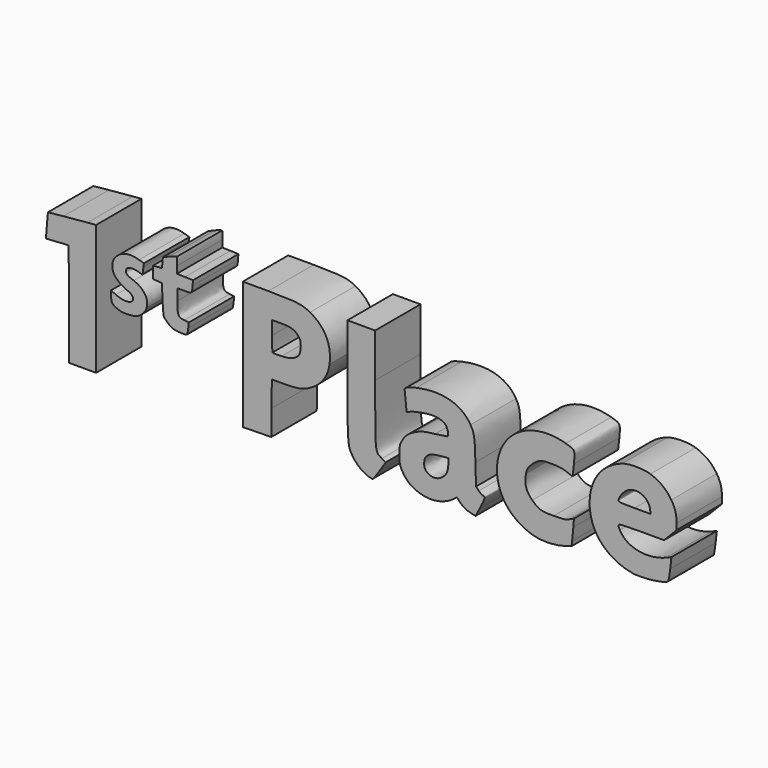
from build123d import *

# Parameters (mm, degrees)
F1_DEPTH = 6.35


# Not quite as in the source:
# - ends of sketch curves that miss each other by under 0.0002 mm in the source are joined


with BuildPart() as f1:
    # F0 (on Front) → F1 (new body)
    with BuildSketch(Plane.XZ):
        with BuildLine():
            add(Edge.make_bspline(
                [(0.3341400629, -8.891573857), (-0.294670775, -8.6645318704), (-0.976808264, -8.1246552902), (-1.3296902624, -7.574737026)],
                knots=[0, 0, 0, 0, 1, 1, 1, 1], degree=3))
            add(Edge.make_bspline(
                [(0.8350588344, -9.0026580356), (0.7635369283, -9.0152123713), (0.5381243175, -8.9652247697), (0.3341400629, -8.891573857)],
                knots=[0, 0, 0, 0, 1, 1, 1, 1], degree=3))
            add(Edge.make_bspline(
                [(1.6370563807, -7.9375592211), (1.2674791345, -8.510809568), (0.9065796253, -8.9901037), (0.8350588344, -9.0026580356)],
                knots=[0, 0, 0, 0, 1, 1, 1, 1], degree=3))
            Line((1.6370563807, -7.9375592211), (1.8985483475, -6.6505150987))
            add(Edge.make_bspline(
                [(1.123237547, 0.7960059272), (1.123237547, -6.5406989559), (1.0841035293, -6.1648384081), (1.8985483475, -6.6505150987)],
                knots=[0, 0, 0, 0, 1, 1, 1, 1], degree=3))
            Line((1.123237547, 0.7960059272), (1.1249048919, 5.7024196408))
            Line((1.1249048919, 5.7024196408), (-1.9611174698, 5.7063939098))
            Line((-1.9611174698, 5.7063939098), (-1.9611174698, 0.6585863056))
            add(Edge.make_bspline(
                [(-1.3296902624, -7.574737026), (-1.9722420587, -6.5734069203), (-1.9611174698, -6.7184604076), (-1.9611174698, 0.6585863056)],
                knots=[0, 0, 0, 0, 1, 1, 1, 1], degree=3))
        make_face()
        Polygon((1.8985483475, -6.6505150987), (1.6370563807, -7.9375592211), (2.3090161255, -6.8952883976), align=None)
    extrude(amount=F1_DEPTH)


with BuildPart() as f1b:
    # F0 (on Front) → F1, piece 2 (new body)
    with BuildSketch(Plane.XZ):
        with BuildLine():
            add(Edge.make_bspline(
                [(6.6803148923, -8.8230898838), (5.4982367035, -8.6125914713), (4.6605144496, -8.0535092224), (4.1522941559, -7.135933052)],
                knots=[0, 0, 0, 0, 1, 1, 1, 1], degree=3))
            add(Edge.make_bspline(
                [(9.910150536, -8.0284407), (9.0040190305, -8.7195815781), (7.78427895, -9.0196789355), (6.6803148923, -8.8230898838)],
                knots=[0, 0, 0, 0, 1, 1, 1, 1], degree=3))
            Line((9.910150536, -8.0284407), (10.2834750122, -7.7436924873))
            Line((10.2834750122, -7.7436924873), (10.5754578323, -8.0633735822))
            add(Edge.make_bspline(
                [(11.9336714428, -8.8088994808), (11.3485816335, -8.6774375088), (10.9229141541, -8.4437876836), (10.5754578323, -8.0633735822)],
                knots=[0, 0, 0, 0, 1, 1, 1, 1], degree=3))
            Line((11.9336714428, -8.8088994808), (12.3629088279, -8.9053426966))
            Line((12.3629088279, -8.9053426966), (12.8352650082, -8.0015967045))
            add(Edge.make_bspline(
                [(13.2301672836, -6.6273569945), (13.4991191377, -6.6273569945), (13.4326637987, -6.8586134996), (12.8352650082, -8.0015967045)],
                knots=[0, 0, 0, 0, 1, 1, 1, 1], degree=3))
            add(Edge.make_bspline(
                [(12.7221990357, -6.3069833312), (12.8910965041, -6.4831890133), (13.1196819926, -6.6273569945), (13.2301672836, -6.6273569945)],
                knots=[0, 0, 0, 0, 1, 1, 1, 1], degree=3))
            Line((12.7221990357, -6.3069833312), (12.4151135405, -5.9866096679))
            Line((12.4151135405, -5.9866096679), (12.3465570762, -3.6147078996))
            add(Edge.make_bspline(
                [(11.7983451399, -0.1012894763), (12.2270594741, -0.8328368689), (12.2750385158, -1.1403271987), (12.3465570762, -3.6147078996)],
                knots=[0, 0, 0, 0, 1, 1, 1, 1], degree=3))
            add(Edge.make_bspline(
                [(5.7503494429, 1.5688051915), (8.5603079697, 2.2020480209), (10.8130600929, 1.5799721598), (11.7983451399, -0.1012894763)],
                knots=[0, 0, 0, 0, 1, 1, 1, 1], degree=3))
            add(Edge.make_bspline(
                [(4.6961912015, 1.2469192532), (4.858749606, 1.3299315493), (5.3331199224, 1.4747798312), (5.7503494429, 1.5688051915)],
                knots=[0, 0, 0, 0, 1, 1, 1, 1], degree=3))
            add(Edge.make_bspline(
                [(4.4566316824, 0.7107497541), (4.4067221482, 1.0541008516), (4.4327698574, 1.1124015044), (4.6961912015, 1.2469192532)],
                knots=[0, 0, 0, 0, 1, 1, 1, 1], degree=3))
            add(Edge.make_bspline(
                [(4.5795397099, -0.4295992373), (4.5427399042, -0.0142890569), (4.4874303439, 0.4988684354), (4.4566316824, 0.7107497541)],
                knots=[0, 0, 0, 0, 1, 1, 1, 1], degree=3))
            Line((4.5795397099, -0.4295992373), (4.6464489543, -1.184710684))
            Line((4.6464489543, -1.184710684), (5.0072993927, -1.03393821))
            add(Edge.make_bspline(
                [(7.5522841514, -0.5632013683), (6.849403068, -0.5632013683), (5.5656132364, -0.8006586468), (5.0072993927, -1.03393821)],
                knots=[0, 0, 0, 0, 1, 1, 1, 1], degree=3))
            add(Edge.make_bspline(
                [(9.0299909029, -1.0454040645), (8.7617907253, -0.7334761668), (8.2399856077, -0.5632013683), (7.5522841514, -0.5632013683)],
                knots=[0, 0, 0, 0, 1, 1, 1, 1], degree=3))
            add(Edge.make_bspline(
                [(9.222734583, -2.0813848949), (9.3763431301, -1.986449493), (9.2485547818, -1.2996045464), (9.0299909029, -1.0454040645)],
                knots=[0, 0, 0, 0, 1, 1, 1, 1], degree=3))
            add(Edge.make_bspline(
                [(7.8341817928, -2.2987833406), (8.5349439069, -2.2181130633), (9.1597933874, -2.1202835954), (9.222734583, -2.0813848949)],
                knots=[0, 0, 0, 0, 1, 1, 1, 1], degree=3))
            add(Edge.make_bspline(
                [(5.5145226556, -2.8919966091), (6.2193665737, -2.5260584139), (6.5136646466, -2.4507959693), (7.8341817928, -2.2987833406)],
                knots=[0, 0, 0, 0, 1, 1, 1, 1], degree=3))
            add(Edge.make_bspline(
                [(4.1460398507, -4.1437375873), (4.462187843, -3.573149335), (4.8030229433, -3.2613887243), (5.5145226556, -2.8919966091)],
                knots=[0, 0, 0, 0, 1, 1, 1, 1], degree=3))
            add(Edge.make_bspline(
                [(3.841652138, -5.6340901247), (3.841652138, -4.7904213738), (3.8731333307, -4.6362819691), (4.1460398507, -4.1437375873)],
                knots=[0, 0, 0, 0, 1, 1, 1, 1], degree=3))
            add(Edge.make_bspline(
                [(4.1522941559, -7.135933052), (3.872362695, -6.6305265265), (3.841652138, -6.4820503461), (3.841652138, -5.6340901247)],
                knots=[0, 0, 0, 0, 1, 1, 1, 1], degree=3))
        make_face()
        with BuildLine():
            add(Edge.make_bspline(
                [(8.4953860954, -6.3921090203), (9.078585561, -5.9951881479), (9.2640165663, -5.6533482101), (9.312943568, -4.8849497105)],
                knots=[0, 0, 0, 0, 1, 1, 1, 1], degree=3))
            add(Edge.make_bspline(
                [(6.6123439327, -5.6718813849), (6.6123439327, -6.5192282205), (7.6983145951, -6.9345919328), (8.4953860954, -6.3921090203)],
                knots=[0, 0, 0, 0, 1, 1, 1, 1], degree=3))
            add(Edge.make_bspline(
                [(8.4887347622, -4.2627634399), (7.0954923584, -4.3789554498), (6.6123439327, -4.7417854516), (6.6123439327, -5.6718813849)],
                knots=[0, 0, 0, 0, 1, 1, 1, 1], degree=3))
            Line((8.4887347622, -4.2627634399), (9.3571731492, -4.1903381837))
            Line((9.3571731492, -4.1903381837), (9.312943568, -4.8849497105))
        make_face(mode=Mode.SUBTRACT)
    extrude(amount=F1_DEPTH)


with BuildPart() as f1c:
    # F0 (on Front) → F1, piece 3 (new body)
    with BuildSketch(Plane.XZ):
        with BuildLine():
            add(Edge.make_bspline(
                [(19.2990995127, -8.8130080508), (18.1354663941, -8.6186316491), (16.9370977921, -7.9656601), (16.108837294, -7.0746892624)],
                knots=[0, 0, 0, 0, 1, 1, 1, 1], degree=3))
            add(Edge.make_bspline(
                [(22.5415642135, -8.5618533085), (21.4959376118, -8.8907418828), (20.3129850692, -8.9823728077), (19.2990995127, -8.8130080508)],
                knots=[0, 0, 0, 0, 1, 1, 1, 1], degree=3))
            Line((22.5415642135, -8.5618533085), (23.1055379359, -8.3844621188))
            Line((23.1055379359, -8.3844621188), (23.167619276, -7.8457108229))
            add(Edge.make_bspline(
                [(23.3004741915, -6.4435865919), (23.2615487251, -6.918443156), (23.2017647938, -7.5493986139), (23.167619276, -7.8457108229)],
                knots=[0, 0, 0, 0, 1, 1, 1, 1], degree=3))
            Line((23.3004741915, -6.4435865919), (23.3712477669, -5.5802136568))
            Line((23.3712477669, -5.5802136568), (22.8595144451, -5.8150668335))
            add(Edge.make_bspline(
                [(21.0931293503, -6.0511133245), (22.1704557332, -6.0501096022), (22.4201082377, -6.0167269134), (22.8595144451, -5.8150668335)],
                knots=[0, 0, 0, 0, 1, 1, 1, 1], degree=3))
            add(Edge.make_bspline(
                [(18.7058996272, -5.2827683568), (19.4276317308, -5.9682292819), (19.6893032524, -6.0524493904), (21.0931293503, -6.0511133245)],
                knots=[0, 0, 0, 0, 1, 1, 1, 1], degree=3))
            add(Edge.make_bspline(
                [(18.0109624482, -2.8942572148), (17.8013506571, -3.9224056654), (18.0028880599, -4.6150866996), (18.7058996272, -5.2827683568)],
                knots=[0, 0, 0, 0, 1, 1, 1, 1], degree=3))
            add(Edge.make_bspline(
                [(18.6761024575, -1.7594264656), (18.21249539, -2.2121732577), (18.1167001327, -2.3756138225), (18.0109624482, -2.8942572148)],
                knots=[0, 0, 0, 0, 1, 1, 1, 1], degree=3))
            add(Edge.make_bspline(
                [(21.1680951392, -1.0013573838), (19.8494014219, -0.9399697273), (19.364021387, -1.0876217402), (18.6761024575, -1.7594264656)],
                knots=[0, 0, 0, 0, 1, 1, 1, 1], degree=3))
            add(Edge.make_bspline(
                [(22.651465115, -1.2766338037), (22.2817964186, -1.1107608852), (21.8677776942, -1.033929288), (21.1680951392, -1.0013573838)],
                knots=[0, 0, 0, 0, 1, 1, 1, 1], degree=3))
            add(Edge.make_bspline(
                [(23.2178656149, -1.4531182976), (23.1883795991, -1.4826020828), (22.9334988166, -1.4031853431), (22.651465115, -1.2766338037)],
                knots=[0, 0, 0, 0, 1, 1, 1, 1], degree=3))
            add(Edge.make_bspline(
                [(23.3722693332, -0.188521867), (23.3168326347, -0.8545652264), (23.2473494001, -1.4236333971), (23.2178656149, -1.4531182976)],
                knots=[0, 0, 0, 0, 1, 1, 1, 1], degree=3))
            add(Edge.make_bspline(
                [(22.4561652889, 1.526791606), (23.5005272005, 1.228131802), (23.491576228, 1.2448906189), (23.3722693332, -0.188521867)],
                knots=[0, 0, 0, 0, 1, 1, 1, 1], degree=3))
            add(Edge.make_bspline(
                [(15.3785177883, -1.0380088616), (16.6014798174, 1.3103377745), (19.5176968489, 2.3671179616), (22.4561652889, 1.526791606)],
                knots=[0, 0, 0, 0, 1, 1, 1, 1], degree=3))
            add(Edge.make_bspline(
                [(16.108837294, -7.0746892624), (14.6279375903, -5.4816626241), (14.3331822661, -3.0452772736), (15.3785177883, -1.0380088616)],
                knots=[0, 0, 0, 0, 1, 1, 1, 1], degree=3))
        make_face()
    extrude(amount=F1_DEPTH)


with BuildPart() as f1d:
    # F0 (on Front) → F1, piece 4 (new body)
    with BuildSketch(Plane.XZ):
        with BuildLine():
            add(Edge.make_bspline(
                [(29.903238362, -8.8266006814), (27.0024117392, -8.2969642993), (25.1184740332, -6.2024088494), (25.1184740332, -3.5069181607)],
                knots=[0, 0, 0, 0, 1, 1, 1, 1], degree=3))
            add(Edge.make_bspline(
                [(33.9080156595, -8.3350767507), (33.5456774816, -8.6974149285), (30.9443493286, -9.0166867278), (29.903238362, -8.8266006814)],
                knots=[0, 0, 0, 0, 1, 1, 1, 1], degree=3))
            add(Edge.make_bspline(
                [(34.137996322, -7.0373151045), (34.0623870356, -7.7002034301), (33.9588965739, -8.2841958363), (33.9080156595, -8.3350767507)],
                knots=[0, 0, 0, 0, 1, 1, 1, 1], degree=3))
            Line((34.137996322, -7.0373151045), (34.2754661296, -5.832063198))
            Line((34.2754661296, -5.832063198), (33.6961767201, -6.0692918508))
            add(Edge.make_bspline(
                [(28.5075714112, -5.0380931997), (29.2647761765, -6.4834421744), (31.5673776107, -6.9410681722), (33.6961767201, -6.0692918508)],
                knots=[0, 0, 0, 0, 1, 1, 1, 1], degree=3))
            add(Edge.make_bspline(
                [(30.9040900267, -4.4317133249), (28.1192279035, -4.4317133249), (28.1816248585, -4.4159258882), (28.5075714112, -5.0380931997)],
                knots=[0, 0, 0, 0, 1, 1, 1, 1], degree=3))
            Line((30.9040900267, -4.4317133249), (33.4485205077, -4.4317133249))
            Line((33.4485205077, -4.4317133249), (34.1452766545, -3.70999795))
            Line((34.1452766545, -3.70999795), (34.8420339165, -2.9882825751))
            Line((34.8420339165, -2.9882825751), (34.8420339165, -2.2845059484))
            add(Edge.make_bspline(
                [(34.2608720072, -0.1972598274), (34.691281517, -0.8734106704), (34.8420339165, -1.4148407896), (34.8420339165, -2.2845059484)],
                knots=[0, 0, 0, 0, 1, 1, 1, 1], degree=3))
            add(Edge.make_bspline(
                [(31.9145105108, 1.5875614157), (32.9791643418, 1.2233529686), (33.7108756757, 0.6667566052), (34.2608720072, -0.1972598274)],
                knots=[0, 0, 0, 0, 1, 1, 1, 1], degree=3))
            add(Edge.make_bspline(
                [(28.7778782904, 1.5911859685), (29.5707598076, 1.8574244266), (31.1309156554, 1.8556210722), (31.9145105108, 1.5875614157)],
                knots=[0, 0, 0, 0, 1, 1, 1, 1], degree=3))
            add(Edge.make_bspline(
                [(25.1184740332, -3.5069181607), (25.1184740332, -1.0660918966), (26.4694764565, 0.8160591837), (28.7778782904, 1.5911859685)],
                knots=[0, 0, 0, 0, 1, 1, 1, 1], degree=3))
        make_face()
        with BuildLine():
            add(Edge.make_bspline(
                [(31.8866059153, -1.9273045982), (31.7402542805, -0.8361681117), (30.5140814552, -0.2657270719), (29.4574819381, -0.7972270318)],
                knots=[0, 0, 0, 0, 1, 1, 1, 1], degree=3))
            Line((31.8866059153, -1.9273045982), (31.942043729, -2.3406262932))
            Line((31.942043729, -2.3406262932), (30.150852195, -2.3406262932))
            add(Edge.make_bspline(
                [(28.359660661, -2.1786020921), (28.359660661, -2.3186258154), (28.6028737293, -2.3406262932), (30.150852195, -2.3406262932)],
                knots=[0, 0, 0, 0, 1, 1, 1, 1], degree=3))
            add(Edge.make_bspline(
                [(29.4574819381, -0.7972270318), (28.9451408067, -1.0549494637), (28.359660661, -1.791651528), (28.359660661, -2.1786020921)],
                knots=[0, 0, 0, 0, 1, 1, 1, 1], degree=3))
        make_face(mode=Mode.SUBTRACT)
    extrude(amount=F1_DEPTH)


with BuildPart() as f1e:
    # F0 (on Front) → F1, piece 5 (new body)
    with BuildSketch(Plane.XZ):
        with BuildLine():
            add(Edge.make_bspline(
                [(-33.1183308593, -2.8695689917), (-33.1183308593, 0.2898075763), (-33.1536179718, 2.8954651182), (-33.1967466648, 2.9207778796)],
                knots=[0, 0, 0, 0, 1, 1, 1, 1], degree=3))
            Line((-33.1183308593, -2.8695689917), (-33.1183308593, -8.6138907341))
            Line((-33.1183308593, -8.6138907341), (-31.6022919528, -8.6138907341))
            Line((-31.6022919528, -8.6138907341), (-30.0862530462, -8.6138907341))
            Line((-30.0862530462, -8.6138907341), (-30.0862530462, -1.3349255345))
            Line((-30.0862530462, -1.3349255345), (-30.0862530462, 5.9440396651))
            Line((-30.0862530462, 5.9440396651), (-31.0533813142, 5.8684638361))
            add(Edge.make_bspline(
                [(-33.7456573034, 5.6207842035), (-32.7968260567, 5.7154419088), (-31.5853018616, 5.8268985799), (-31.0533813142, 5.8684638361)],
                knots=[0, 0, 0, 0, 1, 1, 1, 1], degree=3))
            Line((-33.7456573034, 5.6207842035), (-35.4708050246, 5.4486770541))
            Line((-35.4708050246, 5.4486770541), (-35.5891279928, 4.1417469623))
            add(Edge.make_bspline(
                [(-35.6736415507, 2.7973512623), (-35.6922364824, 2.8179576814), (-35.654205444, 3.4229356906), (-35.5891279928, 4.1417469623)],
                knots=[0, 0, 0, 0, 1, 1, 1, 1], degree=3))
            add(Edge.make_bspline(
                [(-34.4574974448, 2.8633437738), (-35.1077818063, 2.8064405255), (-35.6550466191, 2.7767437281), (-35.6736415507, 2.7973512623)],
                knots=[0, 0, 0, 0, 1, 1, 1, 1], degree=3))
            add(Edge.make_bspline(
                [(-33.1967466648, 2.9207778796), (-33.2398753578, 2.9460917563), (-33.8072130834, 2.9202202561), (-34.4574974448, 2.8633437738)],
                knots=[0, 0, 0, 0, 1, 1, 1, 1], degree=3))
        make_face()
    extrude(amount=F1_DEPTH)


with BuildPart() as f1f:
    # F0 (on Front) → F1, piece 6 (new body)
    with BuildSketch(Plane.XZ):
        with BuildLine():
            add(Edge.make_bspline(
                [(-10.8221040501, 5.7063939098), (-7.6861554761, 5.7023455632), (-7.0627112068, 5.6253366418), (-6.1515767032, 5.1294353665)],
                knots=[0, 0, 0, 0, 1, 1, 1, 1], degree=3))
            Line((-10.8221040501, 5.7063939098), (-13.6712110927, 5.7100630725))
            Line((-13.6712110927, 5.7100630725), (-13.6712110927, -1.454637264))
            Line((-13.6712110927, -1.454637264), (-13.6712110927, -8.6193364852))
            Line((-13.6712110927, -8.6193364852), (-12.0767569382, -8.5904761231))
            Line((-12.0767569382, -8.5904761231), (-10.4823016686, -8.5616135304))
            Line((-10.4823016686, -8.5616135304), (-10.4544829471, -5.7125053726))
            Line((-10.4544829471, -5.7125053726), (-10.4266642257, -2.86339833))
            Line((-10.4266642257, -2.86339833), (-9.0358363316, -2.86339833))
            add(Edge.make_bspline(
                [(-5.9198529096, -2.1731318055), (-6.8391521366, -2.7285359698), (-7.4479509821, -2.86339833), (-9.0358363316, -2.86339833)],
                knots=[0, 0, 0, 0, 1, 1, 1, 1], degree=3))
            add(Edge.make_bspline(
                [(-3.9618338056, 0.7475562512), (-4.106115542, -0.4509182992), (-4.8119598367, -1.5037928913), (-5.9198529096, -2.1731318055)],
                knots=[0, 0, 0, 0, 1, 1, 1, 1], degree=3))
            add(Edge.make_bspline(
                [(-6.1515767032, 5.1294353665), (-4.4820987671, 4.2207912095), (-3.7258765344, 2.707520346), (-3.9618338056, 0.7475562512)],
                knots=[0, 0, 0, 0, 1, 1, 1, 1], degree=3))
        make_face()
        with BuildLine():
            add(Edge.make_bspline(
                [(-7.9490125053, 0.0494261201), (-7.4005150657, 0.3295772847), (-7.1888378371, 0.723029739), (-7.1888378371, 1.4623950131)],
                knots=[0, 0, 0, 0, 1, 1, 1, 1], degree=3))
            add(Edge.make_bspline(
                [(-9.3322031878, -0.224474085), (-8.6457396556, -0.1894285629), (-8.2716032796, -0.1153415886), (-7.9490125053, 0.0494261201)],
                knots=[0, 0, 0, 0, 1, 1, 1, 1], degree=3))
            add(Edge.make_bspline(
                [(-10.351609217, -0.1913233675), (-10.3084803846, -0.2359789731), (-9.8497480617, -0.2508965172), (-9.3322031878, -0.224474085)],
                knots=[0, 0, 0, 0, 1, 1, 1, 1], degree=3))
            add(Edge.make_bspline(
                [(-10.4300244649, 1.4407581058), (-10.4300244649, 0.5877681204), (-10.3947369342, -0.1466677619), (-10.351609217, -0.1913233675)],
                knots=[0, 0, 0, 0, 1, 1, 1, 1], degree=3))
            Line((-10.4300244649, 1.4407581058), (-10.4300244649, 2.9916484815))
            Line((-10.4300244649, 2.9916484815), (-9.4333995864, 2.9916484815))
            add(Edge.make_bspline(
                [(-7.4714804635, 2.3705172345), (-7.8854233511, 2.8624593829), (-8.2934821955, 2.9916484815), (-9.4333995864, 2.9916484815)],
                knots=[0, 0, 0, 0, 1, 1, 1, 1], degree=3))
            add(Edge.make_bspline(
                [(-7.1888378371, 1.4623950131), (-7.1888378371, 1.9316987623), (-7.2396719112, 2.0950289177), (-7.4714804635, 2.3705172345)],
                knots=[0, 0, 0, 0, 1, 1, 1, 1], degree=3))
        make_face(mode=Mode.SUBTRACT)
    extrude(amount=F1_DEPTH)


with BuildPart() as f1g:
    # F0 (on Front) → F1, piece 7 (new body)
    with BuildSketch(Plane.XZ):
        with BuildLine():
            add(Edge.make_bspline(
                [(-27.3678384552, -1.6456735009), (-28.2874499513, -1.3459296768), (-28.4093118771, -1.1987995995), (-28.4119550125, -0.3850406582)],
                knots=[0, 0, 0, 0, 1, 1, 1, 1], degree=3))
            add(Edge.make_bspline(
                [(-25.6661521853, -1.5877587235), (-26.0796188625, -1.7116370159), (-27.062802784, -1.745097772), (-27.3678384552, -1.6456735009)],
                knots=[0, 0, 0, 0, 1, 1, 1, 1], degree=3))
            add(Edge.make_bspline(
                [(-24.4353756204, -0.3788354238), (-24.5977388566, -0.9207551365), (-25.1059145405, -1.4199073568), (-25.6661521853, -1.5877587235)],
                knots=[0, 0, 0, 0, 1, 1, 1, 1], degree=3))
            add(Edge.make_bspline(
                [(-25.8758052406, 1.8415522311), (-24.7249617748, 1.4109653971), (-24.1600389772, 0.5401537645), (-24.4353756204, -0.3788354238)],
                knots=[0, 0, 0, 0, 1, 1, 1, 1], degree=3))
            add(Edge.make_bspline(
                [(-26.7405120111, 2.5302774842), (-26.7405120111, 2.2183540475), (-26.6143731131, 2.1178859052), (-25.8758052406, 1.8415522311)],
                knots=[0, 0, 0, 0, 1, 1, 1, 1], degree=3))
            add(Edge.make_bspline(
                [(-25.250612264, 2.842548878), (-26.0427577182, 3.1252428058), (-26.7405120111, 2.9789982346), (-26.7405120111, 2.5302774842)],
                knots=[0, 0, 0, 0, 1, 1, 1, 1], degree=3))
            add(Edge.make_bspline(
                [(-24.8573817439, 2.9255533673), (-24.8584969909, 2.7128255761), (-24.876471427, 2.7090270448), (-25.250612264, 2.842548878)],
                knots=[0, 0, 0, 0, 1, 1, 1, 1], degree=3))
            add(Edge.make_bspline(
                [(-24.7926806885, 3.5328187482), (-24.8276336451, 3.3214325991), (-24.8567493989, 3.0481636238), (-24.8573817439, 2.9255533673)],
                knots=[0, 0, 0, 0, 1, 1, 1, 1], degree=3))
            Line((-24.7926806885, 3.5328187482), (-24.7291294528, 3.9171574038))
            Line((-24.7291294528, 3.9171574038), (-25.2833023844, 4.0817299444))
            add(Edge.make_bspline(
                [(-27.7953628209, 3.6096681892), (-27.1749620607, 4.2300689494), (-26.3223434526, 4.3902920266), (-25.2833023844, 4.0817299444)],
                knots=[0, 0, 0, 0, 1, 1, 1, 1], degree=3))
            add(Edge.make_bspline(
                [(-28.207262576, 2.0617588689), (-28.3698466311, 2.66554914), (-28.2358218214, 3.1692091887), (-27.7953628209, 3.6096681892)],
                knots=[0, 0, 0, 0, 1, 1, 1, 1], degree=3))
            add(Edge.make_bspline(
                [(-26.6804436918, 0.6879563357), (-27.5450880085, 1.0758950087), (-28.0686485249, 1.5469853837), (-28.207262576, 2.0617588689)],
                knots=[0, 0, 0, 0, 1, 1, 1, 1], degree=3))
            add(Edge.make_bspline(
                [(-26.0676890652, -0.2570303757), (-25.7655240398, 0.0768578509), (-25.9489687903, 0.3597647908), (-26.6804436918, 0.6879563357)],
                knots=[0, 0, 0, 0, 1, 1, 1, 1], degree=3))
            add(Edge.make_bspline(
                [(-27.8644713325, -0.201050552), (-27.1659330209, -0.5262655026), (-26.334779572, -0.5521615382), (-26.0676890652, -0.2570303757)],
                knots=[0, 0, 0, 0, 1, 1, 1, 1], degree=3))
            Line((-27.8644713325, -0.201050552), (-28.4133825287, 0.054504955))
            Line((-28.4133825287, 0.054504955), (-28.4119550125, -0.3850406582))
        make_face()
    extrude(amount=F1_DEPTH)


with BuildPart() as f1h:
    # F0 (on Front) → F1, piece 8 (new body)
    with BuildSketch(Plane.XZ):
        with BuildLine():
            add(Edge.make_bspline(
                [(-21.5650688474, -1.4350144928), (-21.9463918752, -1.2339856427), (-22.3264680567, -0.8970449851), (-22.4895205156, -0.615478572)],
                knots=[0, 0, 0, 0, 1, 1, 1, 1], degree=3))
            add(Edge.make_bspline(
                [(-19.9009452122, -1.5183446343), (-19.9969769018, -1.6737264242), (-21.229317043, -1.6120175765), (-21.5650688474, -1.4350144928)],
                knots=[0, 0, 0, 0, 1, 1, 1, 1], degree=3))
            add(Edge.make_bspline(
                [(-19.7775910859, -0.8537622485), (-19.8147065065, -1.1695611686), (-19.8702168112, -1.4686235768), (-19.9009452122, -1.5183446343)],
                knots=[0, 0, 0, 0, 1, 1, 1, 1], degree=3))
            Line((-19.7775910859, -0.8537622485), (-19.7101074893, -0.2795806703))
            Line((-19.7101074893, -0.2795806703), (-20.2130125157, -0.2228960104))
            add(Edge.make_bspline(
                [(-20.990019607, 1.4433153672), (-20.990019607, -0.0178433491), (-20.9321985104, -0.1418320509), (-20.2130125157, -0.2228960104)],
                knots=[0, 0, 0, 0, 1, 1, 1, 1], degree=3))
            Line((-20.990019607, 1.4433153672), (-20.990019607, 2.6779852594))
            Line((-20.990019607, 2.6779852594), (-20.2025804952, 2.6779852594))
            add(Edge.make_bspline(
                [(-19.2884615906, 3.484440448), (-19.356219538, 2.6532078166), (-19.3281353877, 2.6779852594), (-20.2025804952, 2.6779852594)],
                knots=[0, 0, 0, 0, 1, 1, 1, 1], degree=3))
            Line((-19.2884615906, 3.484440448), (-19.2440290344, 4.0295096183))
            Line((-19.2440290344, 4.0295096183), (-20.1431623649, 4.0594896885))
            Line((-20.1431623649, 4.0594896885), (-21.0422968107, 4.0894697586))
            Line((-21.0422968107, 4.0894697586), (-21.0098788105, 4.8897141366))
            add(Edge.make_bspline(
                [(-21.0729794865, 5.7489941152), (-21.0204435455, 5.7165259289), (-20.9920482413, 5.3298497155), (-21.0098788105, 4.8897141366)],
                knots=[0, 0, 0, 0, 1, 1, 1, 1], degree=3))
            add(Edge.make_bspline(
                [(-21.8895566569, 5.504504089), (-21.4929759348, 5.6714431837), (-21.1255154274, 5.7814634167), (-21.0729794865, 5.7489941152)],
                knots=[0, 0, 0, 0, 1, 1, 1, 1], degree=3))
            Line((-21.8895566569, 5.504504089), (-22.6106129209, 5.2009784623))
            Line((-22.6106129209, 5.2009784623), (-22.6628901246, 4.6452229952))
            Line((-22.6628901246, 4.6452229952), (-22.7151673282, 4.0894697586))
            Line((-22.7151673282, 4.0894697586), (-23.2118013207, 4.0576026905))
            Line((-23.2118013207, 4.0576026905), (-23.708434198, 4.0257356224))
            Line((-23.708434198, 4.0257356224), (-23.708434198, 3.3575889072))
            Line((-23.708434198, 3.3575889072), (-23.708434198, 2.689442192))
            Line((-23.708434198, 2.689442192), (-23.2118013207, 2.6575751239))
            Line((-23.2118013207, 2.6575751239), (-22.7151673282, 2.6257080558))
            Line((-22.7151673282, 2.6257080558), (-22.6628901246, 1.1096691492))
            add(Edge.make_bspline(
                [(-22.4895205156, -0.615478572), (-22.5581617387, -0.4969445434), (-22.633255781, 0.2502966051), (-22.6628901246, 1.1096691492)],
                knots=[0, 0, 0, 0, 1, 1, 1, 1], degree=3))
        make_face()
    extrude(amount=F1_DEPTH)


solid = Compound([f1.part, f1b.part, f1c.part, f1d.part, f1e.part, f1f.part, f1g.part, f1h.part])
